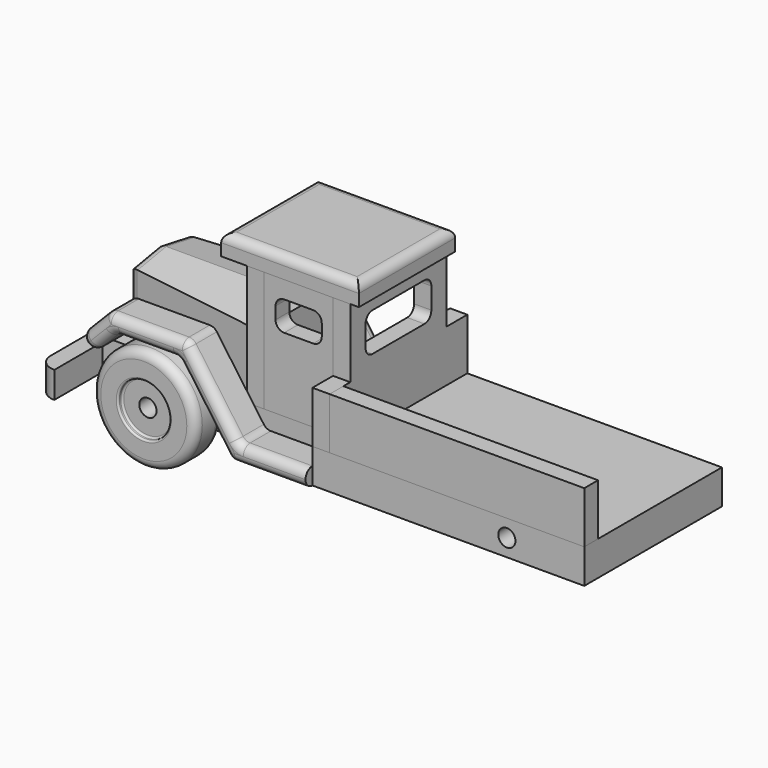
from build123d import *

# Parameters (mm, degrees)
F1_DEPTH       = 20
F2_W           = 18
F2_H           = 10
F3_DEPTH       = 20.001
F5_DEPTH       = 20.001
F6_W           = 10
F6_H           = 70
F7_DEPTH       = 70
F9_DEPTH       = 80
F11_DEPTH      = 70.001
F13_DEPTH      = 208.001
F14_W          = 40
F14_H          = 10
F15_DEPTH      = 70
F16_W          = 10
F16_H          = 100
F17_DEPTH      = 70
F18_W          = 80
F18_H          = 70
F19_DEPTH      = 12
F20_W          = 148
F20_H          = 10
F21_DEPTH      = 30
F22_R          = 5
F23_DEPTH      = 85.001
F23_DEPTH_BACK = 15.001
F24_R          = 30
F24_R_2        = 5
F25_DEPTH      = 20
F26_R          = 5
F27_R          = 15
F28_DEPTH      = 3
F29_R          = 1
F30_R          = 5
F32_DEPTH      = 85.001
F33_R          = 2.4737973705
F34_DEPTH      = 5
F36_DEPTH      = 152.001
F37_W          = 120
F37_H          = 15.3712290645
F38_DEPTH      = 10
F39_R          = 9.99999
F40_R          = 5
F42_DEPTH      = 20
F43_R          = 4.99999
F45_W          = 15
F45_H          = 40
F46_DEPTH      = 162.001


# Not quite as in the source:
# - a fillet or chamfer is up to 0.001 mm smaller than in the source, because OpenCascade refuses the exact size


with BuildPart() as f1:
    # F0 (on Top) → F1 (new body)
    with BuildSketch(Plane.XY):
        Polygon((-8, 50), (-8, 35), (-150, 35), (-150, -35), (-8, -35), (-8, -50), (150, -50), (150, 50), align=None)
    extrude(amount=F1_DEPTH)

    # F2 (on face) → F3 (cut, through all)
    with BuildSketch(Plane.XY.offset(20)):
        with Locations((-141, 30)):
            Rectangle(F2_W, F2_H)
        with Locations((-141, -30)):
            Rectangle(F2_W, F2_H)
    extrude(amount=-F3_DEPTH, mode=Mode.SUBTRACT)

    # F4 (on face) → F5 (cut, through all)
    with BuildSketch(Plane.XY.offset(20)):
        with BuildLine():
            Line((-143, 15), (-150, 15))
            Line((-150, 15), (-150, -15))
            Line((-150, -15), (-143, -15))
            ThreePointArc((-143, -15), (-139.4644660941, -13.5355339059), (-138, -10))
            Line((-138, -10), (-138, 10))
            ThreePointArc((-138, 10), (-139.4644660941, 13.5355339059), (-143, 15))
        make_face()
    extrude(amount=-F5_DEPTH, mode=Mode.SUBTRACT)

    # F22 (on face) → F23 (cut, two sides)
    with BuildSketch(Plane.XZ.offset(35)) as f23_sk:
        with Locations((-102, 10)):
            Circle(F22_R)
        with Locations((105, 10)):
            Circle(F22_R)
    extrude(amount=-F23_DEPTH, mode=Mode.SUBTRACT)
    extrude(f23_sk.sketch, amount=F23_DEPTH_BACK, mode=Mode.SUBTRACT)


with BuildPart() as f7:
    # F6 (on face) → F7 (new body)
    with BuildSketch(Plane.XY.offset(20)):
        with Locations((-53, 0)):
            Rectangle(F6_W, F6_H)
    extrude(amount=F7_DEPTH)

    # F12 (on face) → F13 (cut, through all)
    with BuildSketch(Plane(origin=(-58, 0, 0), x_dir=(0, -1, 0), z_dir=(-1, 0, 0))):
        with BuildLine():
            ThreePointArc((28, 77), (26.5355339059, 80.5355339059), (23, 82))
            Line((23, 82), (-23, 82))
            ThreePointArc((-23, 82), (-26.5355339059, 80.5355339059), (-28, 77))
            Line((-28, 77), (-28, 67))
            ThreePointArc((-28, 67), (-26.5355339059, 63.4644660941), (-23, 62))
            Line((-23, 62), (23, 62))
            ThreePointArc((23, 62), (26.5355339059, 63.4644660941), (28, 67))
            Line((28, 67), (28, 77))
        make_face()
    extrude(amount=-F13_DEPTH, mode=Mode.SUBTRACT)


with BuildPart() as f9:
    # F8 (on face) → F9 (new body)
    with BuildSketch(Plane(origin=(-58, 0, 0), x_dir=(0, -1, 0), z_dir=(-1, 0, 0))):
        Polygon((30, 56), (0, 61.2898094213), (-30, 56), (-30, 20), (0, 20), (30, 20), align=None)
    extrude(amount=F9_DEPTH)

    # F10 (on face) → F11 (cut, through all)
    with BuildSketch(Plane(origin=(0, 0, 20), x_dir=(1, 0, 0), z_dir=(0, 0, -1))):
        Polygon((-138, 20), (-58, 30), (-138, 30), align=None)
        Polygon((-138, -30), (-58, -30), (-138, -20), align=None)
    extrude(amount=-F11_DEPTH, mode=Mode.SUBTRACT)

    # F40
    f40_edges = [f9.edges().sort_by_distance(p)[0] for p in [
        (-138, -20, 38.881635),
        (-138, 0, 20),
        (-138, 20, 38.881635),
        (-138, 10, 59.52654),
        (-138, -10, 59.52654),
    ]]
    fillet(f40_edges, radius=F40_R)


with BuildPart() as f15:
    # F14 (on face) → F15 (new body)
    with BuildSketch(Plane.XY.offset(20)):
        with Locations((-28, -30)):
            Rectangle(F14_W, F14_H)
    extrude(amount=F15_DEPTH)

    # F31 (on face) → F32 (cut, through all)
    with BuildSketch(Plane.XZ.offset(35)):
        with BuildLine():
            ThreePointArc((-14.567978628, 74.8797681928), (-16.032444722, 78.4153020987), (-19.567978628, 79.8797681928))
            Line((-19.567978628, 79.8797681928), (-36.432021372, 79.8797681928))
            ThreePointArc((-36.432021372, 79.8797681928), (-39.967555278, 78.4153020987), (-41.432021372, 74.8797681928))
            Line((-41.432021372, 74.8797681928), (-41.432021372, 67.7844706178))
            ThreePointArc((-41.432021372, 67.7844706178), (-39.967555278, 64.2489367118), (-36.432021372, 62.7844706178))
            Line((-36.432021372, 62.7844706178), (-19.567978628, 62.7844706178))
            ThreePointArc((-19.567978628, 62.7844706178), (-16.032444722, 64.2489367118), (-14.567978628, 67.7844706178))
            Line((-14.567978628, 67.7844706178), (-14.567978628, 74.8797681928))
        make_face()
    extrude(amount=-F32_DEPTH, mode=Mode.SUBTRACT)


with BuildPart() as f17:
    # F16 (on face) → F17 (new body)
    with BuildSketch(Plane.XY.offset(20)):
        with Locations((-3, 0)):
            Rectangle(F16_W, F16_H)
    extrude(amount=F17_DEPTH)

    # F35 (on face) → F36 (cut, through all)
    with BuildSketch(Plane.YZ.offset(2)):
        with BuildLine():
            ThreePointArc((23.8820519298, 75.2886262536), (22.4175858358, 78.8241601595), (18.8820519298, 80.2886262536))
            Line((18.8820519298, 80.2886262536), (-18.8820519298, 80.2886262536))
            ThreePointArc((-18.8820519298, 80.2886262536), (-22.4175858358, 78.8241601595), (-23.8820519298, 75.2886262536))
            Line((-23.8820519298, 75.2886262536), (-23.8820519298, 62.9066798091))
            ThreePointArc((-23.8820519298, 62.9066798091), (-22.4175858358, 59.3711459032), (-18.8820519298, 57.9066798091))
            Line((-18.8820519298, 57.9066798091), (18.8820519298, 57.9066798091))
            ThreePointArc((18.8820519298, 57.9066798091), (22.4175858358, 59.3711459032), (23.8820519298, 62.9066798091))
            Line((23.8820519298, 62.9066798091), (23.8820519298, 75.2886262536))
        make_face()
    extrude(amount=-F36_DEPTH, mode=Mode.SUBTRACT)

    # F45 (on face) → F46 (cut, through all)
    with BuildSketch(Plane.YZ.offset(2)):
        with Locations((-42.5, 70)):
            Rectangle(F45_W, F45_H)
        with Locations((42.5, 70)):
            Rectangle(F45_W, F45_H)
    extrude(amount=-F46_DEPTH, mode=Mode.SUBTRACT)


with BuildPart() as f19:
    # F18 (on face) → F19 (new body)
    with BuildSketch(Plane.XY.offset(90)):
        with Locations((-33, 0)):
            Rectangle(F18_W, F18_H)
    extrude(amount=F19_DEPTH)

    # F30
    f30_edges = [f19.edges().sort_by_distance(p)[0] for p in [
        (7, 0, 102),
        (-33, 35, 102),
        (-73, 0, 102),
        (-33, -35, 102),
    ]]
    fillet(f30_edges, radius=F30_R)

    # F33 (on face) → F34 (cut)
    with BuildSketch(Plane(origin=(0, 0, 90), x_dir=(1, 0, 0), z_dir=(0, 0, -1))):
        with Locations((-3, 0)):
            Circle(F33_R)
    extrude(amount=-F34_DEPTH, mode=Mode.SUBTRACT)


with BuildPart() as f21:
    # F20 (on face) → F21 (new body)
    with BuildSketch(Plane.XY.offset(20)):
        with Locations((76, -45)):
            Rectangle(F20_W, F20_H)
    extrude(amount=F21_DEPTH)


with BuildPart() as f25:
    # F24 (on face) → F25 (new body)
    with BuildSketch(Plane.XZ.offset(35)):
        with Locations((-102, 10)):
            Circle(F24_R)
        with Locations((-102, 10)):
            Circle(F24_R_2, mode=Mode.SUBTRACT)
    extrude(amount=F25_DEPTH)

    # F26
    f26_edges = [f25.edges().sort_by_distance(p)[0] for p in [
        (-132, -55, 10),
        (-132, -35, 10),
    ]]
    fillet(f26_edges, radius=F26_R)

    # F27 (on face) → F28 (cut)
    with BuildSketch(Plane.XZ.offset(55)):
        with Locations((-102, 10)):
            Circle(F27_R)
    extrude(amount=-F28_DEPTH, mode=Mode.SUBTRACT)

    # F29
    f29_edges = [f25.edges().sort_by_distance(p)[0] for p in [
        (-117, -52, 10),
        (-117, -55, 10),
    ]]
    fillet(f29_edges, radius=F29_R)


with BuildPart() as f38:
    # F37 (on face) → F38 (new body)
    with BuildSketch(Plane(origin=(-150, 0, 0), x_dir=(0, -1, 0), z_dir=(-1, 0, 0))):
        with Locations((0, 9.3460926014)):
            Rectangle(F37_W, F37_H)
    extrude(amount=F38_DEPTH)

    # F39 (radius 10 in the source; OpenCascade refuses exactly that, so slightly less here)
    f39_edges = [f38.edges().sort_by_distance(p)[0] for p in [
        (-160, 60, 9.346093),
        (-160, -60, 9.346093),
    ]]
    fillet(f39_edges, radius=F39_R)


with BuildPart() as f42:
    # F41 (on face) → F42 (new body)
    with BuildSketch(Plane.XZ.offset(35)):
        with BuildLine():
            ThreePointArc((-136.1104988043, 32.1548946818), (-132.5609139187, 30.7248219283), (-129.0397642341, 32.2235433298))
            Line((-129.0397642341, 32.2235433298), (-120.2696660562, 41.1656060879))
            ThreePointArc((-120.2696660562, 41.1656060879), (-118.6357927746, 42.2746181593), (-116.699974447, 42.6645631268))
            Line((-116.699974447, 42.6645631268), (-84.80352508, 42.6645631268))
            ThreePointArc((-84.80352508, 42.6645631268), (-82.5096065725, 42.1073030337), (-80.7270117613, 40.559738279))
            Line((-80.7270117613, 40.559738279), (-53.4159983678, 2.1048248478))
            ThreePointArc((-53.4159983678, 2.1048248478), (-51.6334035567, 0.5572600931), (-49.3394850491, 0))
            Line((-49.3394850491, 0), (-8, 0))
            Line((-8, 0), (-8, 10))
            Line((-8, 10), (-44.1761881745, 10))
            ThreePointArc((-44.1761881745, 10), (-46.4701066821, 10.5572600931), (-48.2527014933, 12.1048248478))
            Line((-48.2527014933, 12.1048248478), (-75.5637148867, 50.559738279))
            ThreePointArc((-75.5637148867, 50.559738279), (-77.3463096979, 52.1073030337), (-79.6402282055, 52.6645631268))
            Line((-79.6402282055, 52.6645631268), (-120.8990963965, 52.6645631268))
            ThreePointArc((-120.8990963965, 52.6645631268), (-122.834914724, 52.2746181593), (-124.4687880057, 51.1656060879))
            Line((-124.4687880057, 51.1656060879), (-136.1791474524, 39.225629252))
            ThreePointArc((-136.1791474524, 39.225629252), (-137.6092202058, 35.6760443664), (-136.1104988043, 32.1548946818))
        make_face()
    extrude(amount=F42_DEPTH)

    # F43 (radius 5 in the source; OpenCascade refuses exactly that, so slightly less here)
    f43_edges = [f42.edges().sort_by_distance(p)[0] for p in [
        (-130.323968, -55, 45.195618),
        (-136.110499, -55, 32.154895),
        (-124.654715, -55, 36.694575),
        (-118.635793, -55, 42.274618),
        (-100.75175, -55, 42.664563),
        (-82.509607, -55, 42.107303),
        (-67.071505, -55, 21.332282),
        (-51.633404, -55, 0.55726),
        (-28.669743, -55, 0),
        (-26.088094, -55, 10),
        (-46.470107, -55, 10.55726),
        (-61.908208, -55, 31.332282),
        (-77.34631, -55, 52.107303),
        (-100.269662, -55, 52.664563),
        (-122.834915, -55, 52.274618),
    ]]
    fillet(f43_edges, radius=F43_R)


with BuildPart() as f44_1:
    # F44: instance of F42
    add(f42.part.mirror(Plane.XZ))


solid = Compound([f1.part, f7.part, f9.part, f15.part, f17.part, f19.part, f21.part, f25.part, f38.part, f42.part, f44_1.part])
